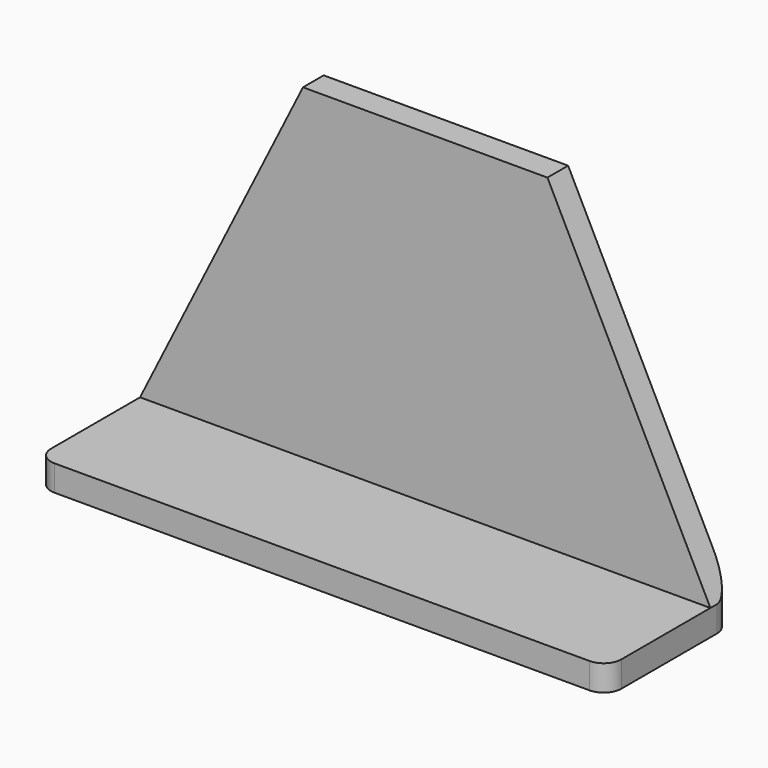
from build123d import *

# Parameters (mm, degrees)
F0_W     = 140
F0_H     = 31.65
F1_DEPTH = 6.35
F2_W     = 140
F2_H     = 6.35
F3_DEPTH = 6.35
F4_R     = 4.33


with BuildPart() as f1:
    # F0 (on Top) → F1 (new body)
    with BuildSketch(Plane.XY):
        Rectangle(F0_W, F0_H)
    extrude(amount=F1_DEPTH)

    # F2 (on face) → F3 (join)
    with BuildSketch(Plane(origin=(0, 15.825, 0), x_dir=(-1, 0, 0), z_dir=(0, 1, 0))):
        with Locations((0, 3.175)):
            Rectangle(F2_W, F2_H)
        Polygon((-30, 86.35), (-70, 6.35), (70, 6.35), (30, 86.35), align=None)
    extrude(amount=F3_DEPTH)

    # F4
    f4_edges = [f1.edges().sort_by_distance(p)[0] for p in [
        (-70, -15.825, 3.175),
        (70, -15.825, 3.175),
        (70, 22.175, 3.175),
        (-70, 22.175, 3.175),
    ]]
    fillet(f4_edges, radius=F4_R)


solid = f1.part
